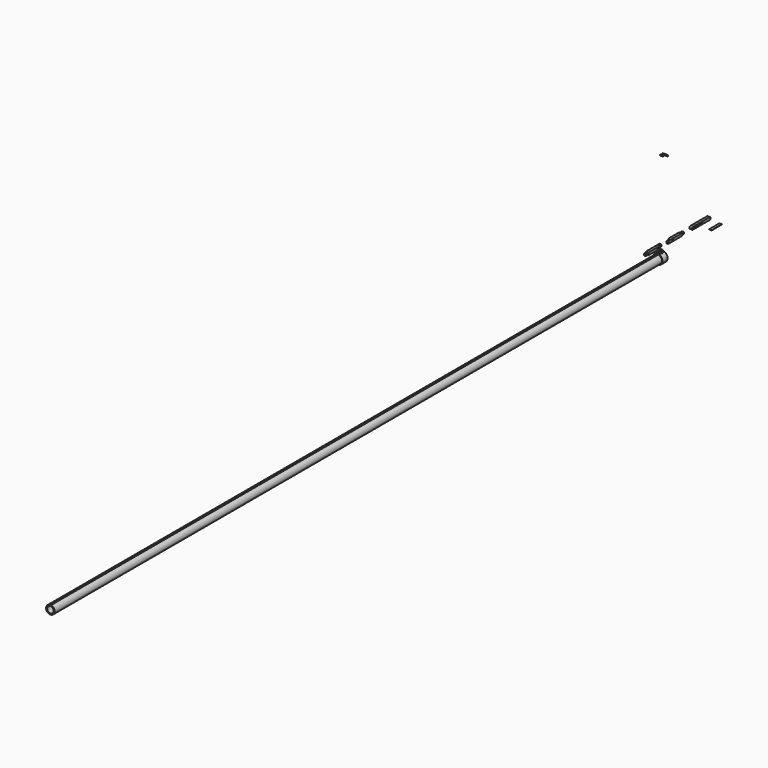
from build123d import *

# Parameters (mm, degrees)
F0_W           = 8.516
F0_H           = 1.016
F0_R           = 0.254
F1_DEPTH       = 1.016
F0_W_2         = 9.398
F2_W           = 0.254
F2_H           = 1.27
F2_W_2         = 0.508
F2_H_2         = 1.778
F3_DEPTH       = 1.017
F4_R           = 0.50799
F4_2_R         = 0.50799
F4_3_R         = 0.50799
F5_R           = 0.127
F5_2_R         = 0.127
F7_DEPTH       = 304.8
F9_DEPTH       = 2.54
F10_W          = 0.508
F10_H          = 1.524
F11_DEPTH      = 304.801
F12_R          = 0.254
F13_DEPTH      = 1.9695
F13_DEPTH_BACK = 1.9695
F14_R          = 0.254
F15_R          = 0.2286
F16_DEPTH      = 2.032
F17_R          = 0.2286
F18_DEPTH      = 1.016
F19_W          = 1.016
F19_H          = 5.08
F20_DEPTH      = 0.1


# Not quite as in the source:
# - a fillet or chamfer is up to 0.001 mm smaller than in the source, because OpenCascade refuses the exact size


with BuildPart() as f1:
    # F0 (on Right) → F1 (new body)
    with BuildSketch(Plane.YZ):
        with Locations((-5.428305112, 4.5706343557)):
            Rectangle(F0_W, F0_H)
        with Locations((-9.178305112, 4.5706343557)):
            Circle(F0_R, mode=Mode.SUBTRACT)
        with Locations((-3.710305112, 4.5706343557)):
            Circle(F0_R, mode=Mode.SUBTRACT)
        with Locations((-1.678305112, 4.5706343557)):
            Circle(F0_R, mode=Mode.SUBTRACT)
    extrude(amount=F1_DEPTH)


with BuildPart() as f1b:
    # F0 (on Right) → F1, piece 2 (new body)
    with BuildSketch(Plane.YZ):
        with Locations((5.428305112, 4.5706343557)):
            Rectangle(F0_W, F0_H)
        with Locations((1.678305112, 4.5706343557)):
            Circle(F0_R, mode=Mode.SUBTRACT)
        with Locations((3.710305112, 4.5706343557)):
            Circle(F0_R, mode=Mode.SUBTRACT)
        with Locations((9.178305112, 4.5706343557)):
            Circle(F0_R, mode=Mode.SUBTRACT)
    extrude(amount=F1_DEPTH)


with BuildPart() as f1c:
    # F0 (on Right) → F1, piece 3 (new body)
    with BuildSketch(Plane.YZ):
        with Locations((17.9813661472, 4.5706343557)):
            Rectangle(F0_W_2, F0_H)
        with Locations((13.7903661472, 4.5706343557)):
            Circle(F0_R, mode=Mode.SUBTRACT)
        with BuildLine():
            ThreePointArc((14.8063661472, 4.5706343557), (14.8807610248, 4.7502394781), (15.0603661472, 4.8246343557))
            Line((15.0603661472, 4.8246343557), (18.2353661472, 4.8246343557))
            ThreePointArc((18.2353661472, 4.8246343557), (18.4149712697, 4.7502394781), (18.4893661472, 4.5706343557))
            ThreePointArc((18.4893661472, 4.5706343557), (18.4149712697, 4.3910292332), (18.2353661472, 4.3166343557))
            Line((18.2353661472, 4.3166343557), (15.0603661472, 4.3166343557))
            ThreePointArc((15.0603661472, 4.3166343557), (14.8807610248, 4.3910292332), (14.8063661472, 4.5706343557))
        make_face(mode=Mode.SUBTRACT)
    extrude(amount=F1_DEPTH)

    # F4#3 (radius 0.508 in the source; OpenCascade refuses exactly that, so slightly less here)
    f4_3_edges = [f1c.edges().sort_by_distance(p)[0] for p in [
        (0.508, 13.282366, 5.078634),
        (0.508, 13.282366, 4.062634),
        (0.508, 22.680366, 5.078634),
        (0.508, 22.680366, 4.062634),
    ]]
    fillet(f4_3_edges, radius=F4_3_R)


with BuildPart() as f3_tool:
    # F2 (on face) → F3 (new body, through all)
    with BuildSketch(Plane.XY.offset(5.0786343557)):
        with Locations((0.127, -9.051305112)):
            Rectangle(F2_W, F2_H)
        with Locations((0.889, -9.051305112)):
            Rectangle(F2_W, F2_H)
        with Locations((0.762, -2.059305112)):
            Rectangle(F2_W_2, F2_H_2)
        with Locations((0.254, 2.059305112)):
            Rectangle(F2_W_2, F2_H_2)
        with Locations((0.127, 9.051305112)):
            Rectangle(F2_W, F2_H)
        with Locations((0.889, 9.051305112)):
            Rectangle(F2_W, F2_H)
    extrude(amount=-F3_DEPTH)


with BuildPart() as f1_1:
    add(f1.part)

    # F3: cut by f3_tool
    add(f3_tool.part, mode=Mode.SUBTRACT)

    # F4 (radius 0.508 in the source; OpenCascade refuses exactly that, so slightly less here)
    f4_edges = [f1_1.edges().sort_by_distance(p)[0] for p in [
        (0.508, -9.686305, 5.078634),
        (0.508, -9.686305, 4.062634),
        (0.254, -1.170305, 5.078634),
        (0.254, -1.170305, 4.062634),
    ]]
    fillet(f4_edges, radius=F4_R)

    # F5
    f5_edges = [f1_1.edges().sort_by_distance(p)[0] for p in [
        (0.762, -2.948305, 5.078634),
        (0.762, -2.948305, 4.062634),
        (0.127, -8.416305, 4.062634),
        (0.127, -8.416305, 5.078634),
        (0.889, -8.416305, 5.078634),
        (0.889, -8.416305, 4.062634),
    ]]
    fillet(f5_edges, radius=F5_R)


with BuildPart() as f1b_1:
    add(f1b.part)

    # F3: cut by f3_tool
    add(f3_tool.part, mode=Mode.SUBTRACT)

    # F4#2 (radius 0.508 in the source; OpenCascade refuses exactly that, so slightly less here)
    f4_2_edges = [f1b_1.edges().sort_by_distance(p)[0] for p in [
        (0.762, 1.170305, 5.078634),
        (0.762, 1.170305, 4.062634),
        (0.508, 9.686305, 5.078634),
        (0.508, 9.686305, 4.062634),
    ]]
    fillet(f4_2_edges, radius=F4_2_R)

    # F5#2
    f5_2_edges = [f1b_1.edges().sort_by_distance(p)[0] for p in [
        (0.254, 2.948305, 5.078634),
        (0.254, 2.948305, 4.062634),
        (0.127, 8.416305, 5.078634),
        (0.127, 8.416305, 4.062634),
        (0.889, 8.416305, 5.078634),
        (0.889, 8.416305, 4.062634),
    ]]
    fillet(f5_2_edges, radius=F5_2_R)


with BuildPart() as f7:
    # F6 (on Front) → F7 (new body)
    with BuildSketch(Plane.XZ):
        with BuildLine():
            Line((-0.254, 1.2443407893), (-0.254, 1.6955808002))
            ThreePointArc((-0.254, 1.6955808002), (0, -1.7145), (0.254, 1.6955808002))
            Line((0.254, 1.6955808002), (0.254, 1.2443407893))
            ThreePointArc((0.254, 1.2443407893), (0, -1.27), (-0.254, 1.2443407893))
        make_face()
    extrude(amount=F7_DEPTH)


with BuildPart() as f9:
    # F8 (on Front) → F9 (new body)
    with BuildSketch(Plane.XZ):
        with BuildLine():
            Line((-0.762, 3.3390339529), (-0.762, 1.8150339529))
            ThreePointArc((-0.762, 1.8150339529), (0, -1.9685), (0.762, 1.8150339529))
            Line((0.762, 1.8150339529), (0.762, 3.3390339529))
            Line((0.762, 3.3390339529), (0, 3.3390339529))
            Line((0, 3.3390339529), (-0.762, 3.3390339529))
        make_face()
        with BuildLine():
            ThreePointArc((0.1905, 1.7677651852), (0, -1.778), (-0.1905, 1.7677651852))
            Line((-0.1905, 1.7677651852), (-0.1905, 1.27))
            Line((-0.1905, 1.27), (0.1905, 1.27))
            Line((0.1905, 1.27), (0.1905, 1.7677651852))
        make_face(mode=Mode.SUBTRACT)
    extrude(amount=F9_DEPTH)

    # F10 (on Front) → F11 (cut, through all)
    with BuildSketch(Plane.XZ):
        with Locations((0, 2.7305)):
            Rectangle(F10_W, F10_H)
    extrude(amount=F11_DEPTH, mode=Mode.SUBTRACT)

    # F12 (on Right) → F13 (cut, two sides)
    with BuildSketch(Plane.YZ) as f13_sk:
        with Locations((-1.27, 2.5770339529)):
            Circle(F12_R)
        with BuildLine():
            Line((0, 1.9685), (0, 3.3390339529))
            Line((0, 3.3390339529), (-0.6516448254, 3.5353413116))
            Line((-0.6516448254, 3.5353413116), (-2.2018356164, 3.5353413116))
            Line((-2.2018356164, 3.5353413116), (-2.54, 3.3390339529))
            Line((-2.54, 3.3390339529), (-2.54, 1.9685))
            Line((-2.54, 1.9685), (-1.778, 1.9685))
            Line((-1.778, 1.9685), (-1.778, 2.5770339529))
            ThreePointArc((-1.778, 2.5770339529), (-1.27, 3.0850339529), (-0.762, 2.5770339529))
            Line((-0.762, 2.5770339529), (-0.762, 1.9685))
            Line((-0.762, 1.9685), (0, 1.9685))
        make_face()
    extrude(amount=-F13_DEPTH, mode=Mode.SUBTRACT)
    extrude(f13_sk.sketch, amount=F13_DEPTH_BACK, mode=Mode.SUBTRACT)

    # F14 (call 1 of 2: OpenCascade refuses the feature's edges together)
    f14_edges = [f9.edges().sort_by_distance(p)[0] for p in [
        (0.762, -1.27, 1.815034),
    ]]
    fillet(f14_edges, radius=F14_R)

    # F14#2 (call 2 of 2)
    f14_2_edges = [f9.edges().sort_by_distance(p)[0] for p in [
        (-0.762, -1.27, 1.815034),
    ]]
    fillet(f14_2_edges, radius=F14_R)


with BuildPart() as f16:
    # F15 (on Right) → F16 (new body)
    with BuildSketch(Plane.YZ):
        with Locations((0, 35.941991955)):
            Circle(F15_R)
    extrude(amount=F16_DEPTH)


with BuildPart() as f18:
    # F17 (on Right) → F18 (new body)
    with BuildSketch(Plane.YZ):
        with Locations((-1.0384203633, 35.9487757087)):
            Circle(F17_R)
    extrude(amount=F18_DEPTH)


with BuildPart() as f20:
    # F19 (on Top) → F20 (new body)
    with BuildSketch(Plane.XY):
        with Locations((0.508, 25.7052464718)):
            Rectangle(F19_W, F19_H)
    extrude(amount=F20_DEPTH)


solid = Compound([f1c.part, f1_1.part, f1b_1.part, f7.part, f9.part, f16.part, f18.part, f20.part])
